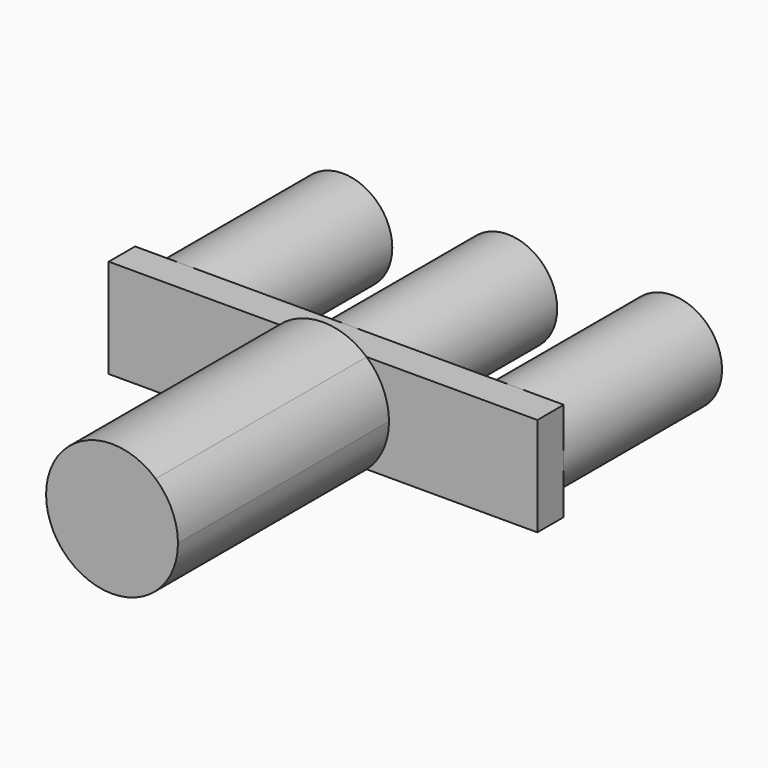
from build123d import *

# Parameters (mm, degrees)
F1_DEPTH = 76.2
F0_R     = 19.05
F3_DEPTH = 12.7
F5_DEPTH = 101.6


with BuildPart() as f1:
    # F0 (on Front) → F1 (new body)
    with BuildSketch(Plane.XZ):
        with BuildLine():
            ThreePointArc((-19.05, 0), (0, -19.05), (19.05, 0))
            ThreePointArc((19.05, 0), (0, 19.05), (-19.05, 0))
        make_face()
    extrude(amount=F1_DEPTH)


with BuildPart() as f1b:
    # F0 (on Front) → F1, piece 2 (new body)
    with BuildSketch(Plane.XZ):
        with Locations((-63.5, 0)):
            Circle(F0_R)
    extrude(amount=F1_DEPTH)


with BuildPart() as f1c:
    # F0 (on Front) → F1, piece 3 (new body)
    with BuildSketch(Plane.XZ):
        with BuildLine():
            ThreePointArc((82.55, 0), (63.5, 19.05), (44.45, 0))
            ThreePointArc((44.45, 0), (63.5, -19.05), (82.55, 0))
        make_face()
    extrude(amount=F1_DEPTH)


with BuildPart() as f3:
    # F2 (on face) → F3 (new body)
    with BuildSketch(Plane.XZ.offset(76.2)):
        with BuildLine():
            ThreePointArc((-9.66e-08, -19.05), (-19.05, 1.085e-07), (1.205e-07, 19.05))
            Line((1.205e-07, 19.05), (-82.55, 19.05))
            Line((-82.55, 19.05), (-82.55, -19.05))
            Line((-82.55, -19.05), (-9.66e-08, -19.05))
        make_face()
        with BuildLine():
            Line((82.55, -19.05), (82.55, 19.05))
            Line((82.55, 19.05), (1.205e-07, 19.05))
            ThreePointArc((1.205e-07, 19.05), (13.4703842242, 13.470384139), (19.05, 0))
            ThreePointArc((19.05, 0), (13.4703841474, -13.4703842158), (-9.66e-08, -19.05))
            Line((-9.66e-08, -19.05), (82.55, -19.05))
        make_face()
        with BuildLine():
            ThreePointArc((19.05, 0), (13.4703842242, 13.470384139), (1.205e-07, 19.05))
            ThreePointArc((1.205e-07, 19.05), (-19.05, 1.085e-07), (-9.66e-08, -19.05))
            ThreePointArc((-9.66e-08, -19.05), (13.4703841474, -13.4703842158), (19.05, 0))
        make_face()
    extrude(amount=F3_DEPTH)

    # F4 (on face) → F5 (join)
    with BuildSketch(Plane.XZ.offset(88.9)):
        with BuildLine():
            Line((-16.8005208253, 19.05), (16.8005208253, 19.05))
            ThreePointArc((16.8005208253, 19.05), (0, 25.4), (-16.8005208253, 19.05))
        make_face()
        with BuildLine():
            ThreePointArc((16.8005208253, -19.05), (23.1505208253, -10.4505208253), (25.4, 0))
            ThreePointArc((25.4, 0), (23.1505208253, 10.4505208253), (16.8005208253, 19.05))
            Line((16.8005208253, 19.05), (-16.8005208253, 19.05))
            ThreePointArc((-16.8005208253, 19.05), (-25.4, 0), (-16.8005208253, -19.05))
            Line((-16.8005208253, -19.05), (16.8005208253, -19.05))
        make_face()
        with BuildLine():
            ThreePointArc((-16.8005208253, -19.05), (0, -25.4), (16.8005208253, -19.05))
            Line((16.8005208253, -19.05), (-16.8005208253, -19.05))
        make_face()
    extrude(amount=F5_DEPTH)


solid = Compound([f1.part, f1b.part, f1c.part, f3.part])
